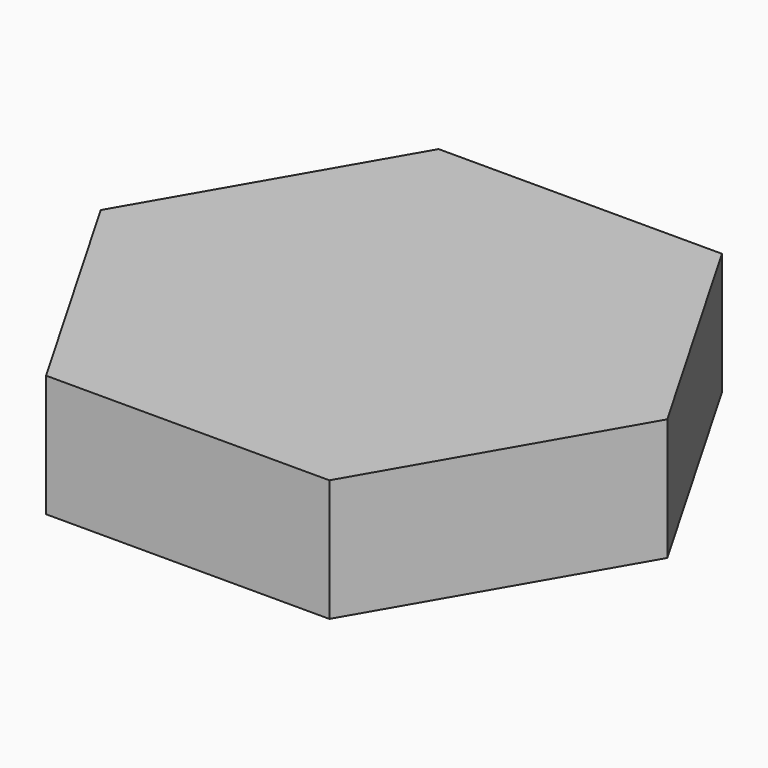
from build123d import *

# Parameters (mm, degrees)
F1_DEPTH = 7.112


# Not quite as in the source:
# - the program builds the solid bodies; features that only make, move or delete a surface that nothing else refers to are left out


with BuildPart() as f1:
    # F0 (on Top) → F1 (new body)
    with BuildSketch(Plane.XY):
        Polygon((-8.255, -14.2980794165), (8.255, -14.2980794165), (16.51, 0), (8.255, 14.2980794165), (-8.255, 14.2980794165), (-16.51, 0), align=None)
    extrude(amount=F1_DEPTH)


solid = f1.part
